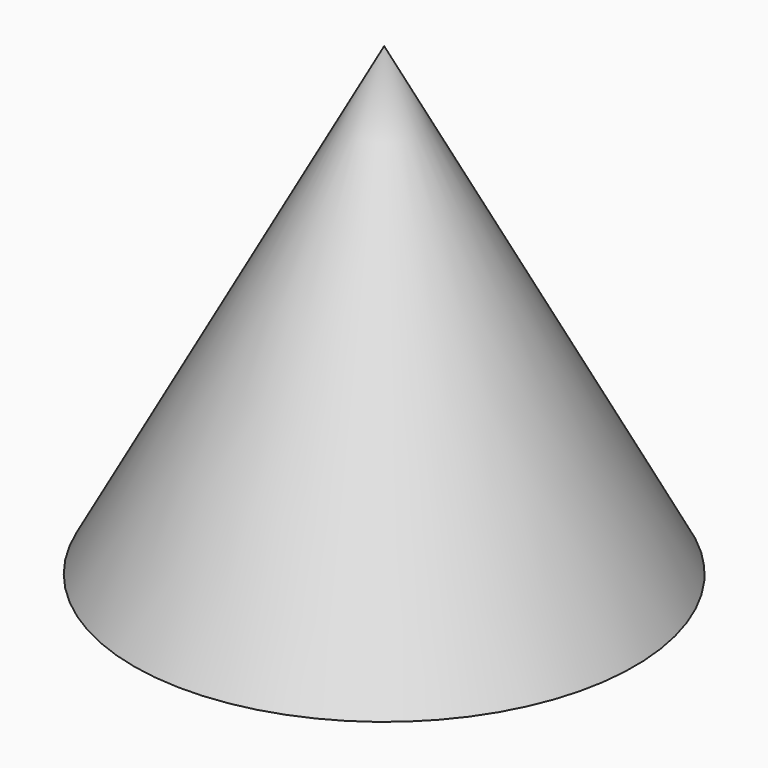
from build123d import *


# Not quite as in the source:
# - the program builds the solid bodies; features that only make, move or delete a surface that nothing else refers to are left out


with BuildPart() as f1:
    # F0 (on Front) → F1 (revolve)
    with BuildSketch(Plane.XZ):
        Polygon((0, 0), (0, 56.3204027712), (-30.3263701499, 0), align=None)
    revolve(axis=Axis((0, 0, 28.1602013856), (0, 0, 1)))


solid = f1.part
